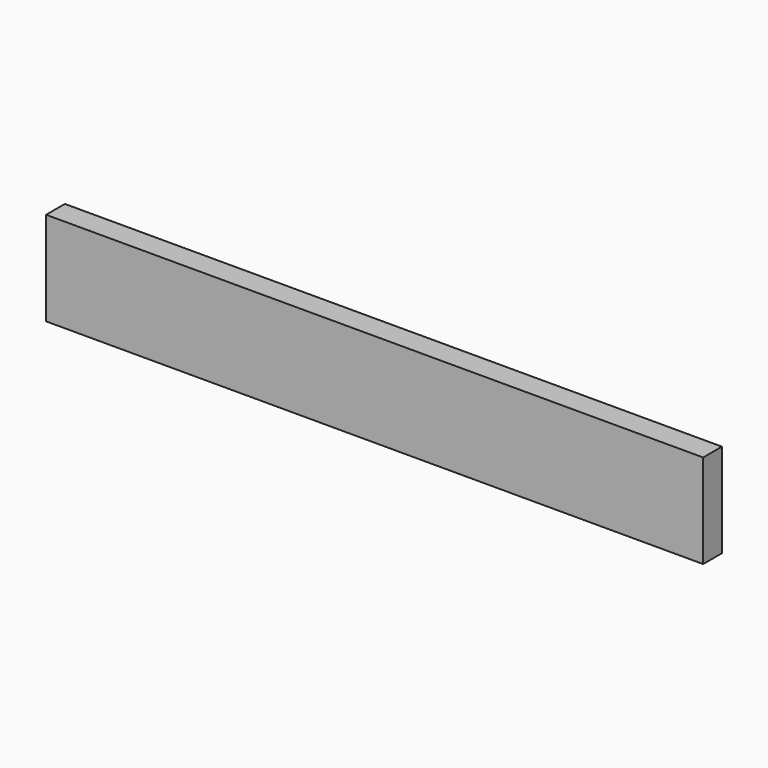
from build123d import *

# Parameters (mm, degrees)
F0_W     = 533.4
F0_H     = 76.2
F1_DEPTH = 19.05


# Not quite as in the source:
# - a feature names something its author has since deleted; it is built from what else it names


with BuildPart() as f1:
    # F0 (on Front) → F1 (new body)
    with BuildSketch(Plane.XZ):
        with Locations((266.7, 38.1)):
            Rectangle(F0_W, F0_H)
    extrude(amount=-F1_DEPTH)


solid = f1.part
